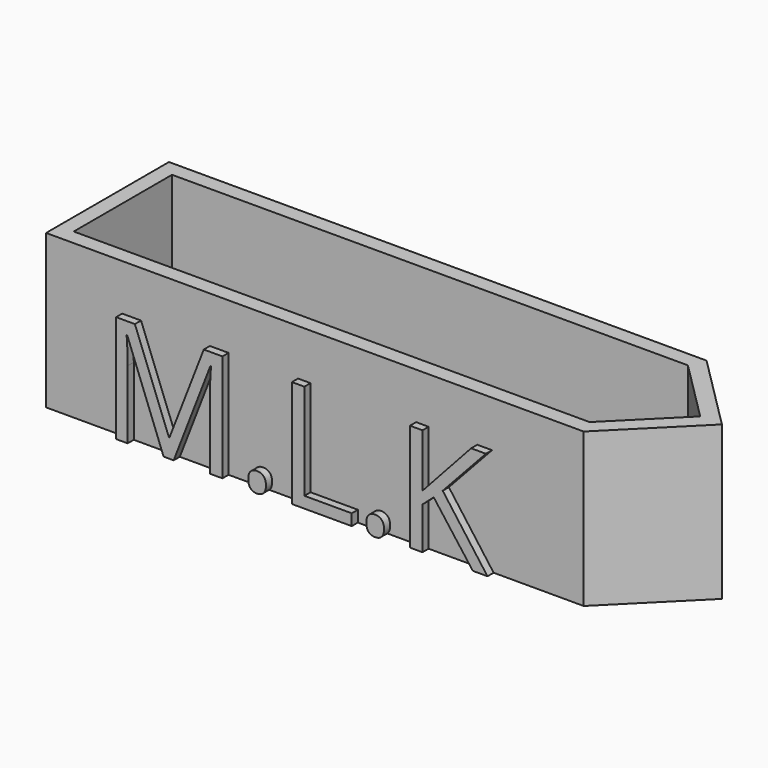
from build123d import *

# Parameters (mm, degrees)
F1_DEPTH     = 25.4
F2_T         = -2.54
F4_TEXT_SIZE = 24.8684806542
F5_DEPTH     = 1.27


# Not quite as in the source:
# - Text() gives the source's letters only with a copy of the font that has no kerning and outlines rounded to 1/6400 em; it was checked with that copy


with BuildPart() as f1:
    # F0 (on Top) → F1 (new body)
    with BuildSketch(Plane.XY):
        Polygon((-50.955273211, 31.3861494228), (-50.955273211, 18.6861494228), (50.644726789, 18.6861494228), (37.944726789, 31.3861494228), align=None)
        Polygon((-50.955273211, 18.6861494228), (-50.955273211, 5.9861494228), (37.944726789, 5.9861494228), (50.644726789, 18.6861494228), align=None)
    extrude(amount=F1_DEPTH)

    # F2
    f2_openings = [f1.faces().sort_by_distance(p)[0] for p in [
        (-3.259718, 18.686149, 25.4),
    ]]
    offset(amount=F2_T, openings=f2_openings)

    # F4 (on face) → F5 (join)
    with BuildSketch(Plane.XZ.offset(-5.9861494228)):
        with Locations((-40.80099985, 0)):
            Text('M.L.K', F4_TEXT_SIZE, font='Open Sans', text_align=(TextAlign.LEFT, TextAlign.BOTTOM))
    extrude(amount=F5_DEPTH)


solid = f1.part
